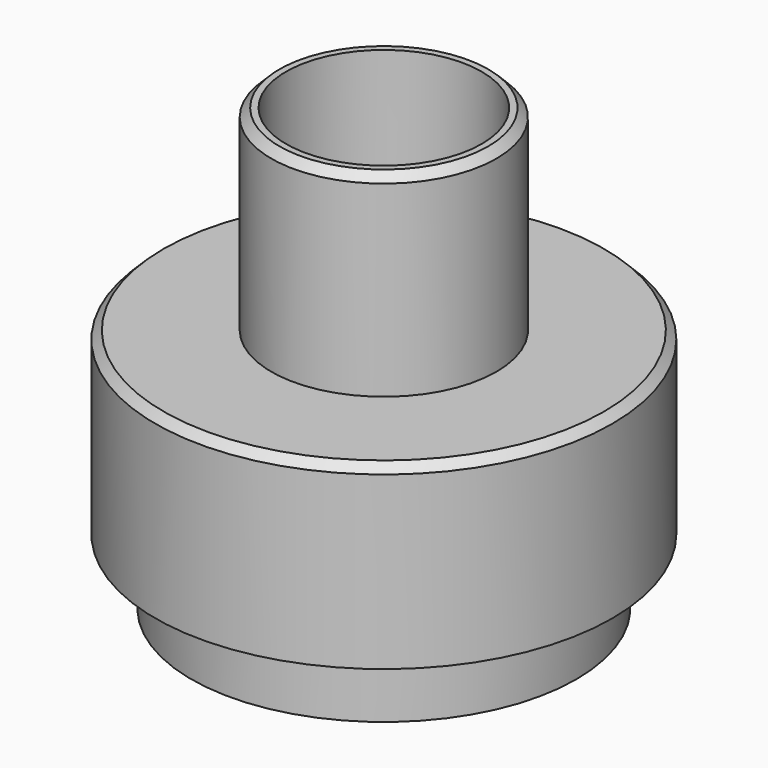
from build123d import *

# Parameters (mm, degrees)
F0_R        = 7
F1_DEPTH    = 5.5
F2_R        = 3.45
F3_DEPTH    = 6
F4_R        = 3
F5_DEPTH    = 25
F6_R        = 6
F6_R_2      = 3
F7_DEPTH    = 2
F8_S5_R     = 6
F8_T6_DEPTH = 11
F9_SIZE     = 0.25
F10_R       = 5.9
F11_DEPTH   = 2
F12_W       = 0.6
F12_H       = 0.6
F13_DEPTH   = 25


# Not quite as in the source:
# - a fillet or chamfer that OpenCascade refuses, or shapes differently, is made with other operations: its cross-section is extruded or revolved along the edge and cut away or added


with BuildPart() as f1:
    # F0 (on Top) → F1 (new body)
    with BuildSketch(Plane.XY):
        Circle(F0_R)
    extrude(amount=F1_DEPTH)

    # F2 (on face) → F3 (join)
    with BuildSketch(Plane.XY.offset(5.5)):
        Circle(F2_R)
    extrude(amount=F3_DEPTH)

    # F4 (on face) → F5 (cut)
    with BuildSketch(Plane.XY.offset(11.5)):
        Circle(F4_R)
    extrude(amount=-F5_DEPTH, mode=Mode.SUBTRACT)

    # F6 (on face) → F7 (cut)
    with BuildSketch(Plane(origin=(0, 0, 0), x_dir=(1, 0, 0), z_dir=(0, 0, -1))):
        Circle(F6_R)
        Circle(F6_R_2, mode=Mode.SUBTRACT)
    extrude(amount=-F7_DEPTH, mode=Mode.SUBTRACT)

    # F8: chamfer of 3.3 on 1 edges, made by hand


with BuildPart() as f8_tool2:
    # F8_s3 → F8_t4 (revolve)
    with BuildSketch(Plane.XZ):
        Polygon((6.3, 2), (3, 5.3), (3, 2), align=None)
    revolve(axis=Axis((0, 0, 2), (0, 0, -1)))

    # F8_s5 → F8_t6 (intersect, symmetric)
    with BuildSketch(Plane.XY.offset(3.6)):
        Circle(F8_S5_R)
    extrude(amount=F8_T6_DEPTH, both=True, mode=Mode.INTERSECT)


with BuildPart() as f1_1:
    add(f1.part)

    # F8_t1: cut F8_tool2
    add(f8_tool2.part, mode=Mode.SUBTRACT)

    # F9
    f9_edges = [f1_1.edges().sort_by_distance(p)[0] for p in [
        (-3.45, 0, 11.5),
        (-7, 0, 5.5),
    ]]
    chamfer(f9_edges, length=F9_SIZE)


with BuildPart() as f11:
    # F10 (on Top) → F11 (new body)
    with BuildSketch(Plane.XY):
        Circle(F10_R)
    extrude(amount=-F11_DEPTH)

    # F12 (on face) → F13 (cut)
    with BuildSketch(Plane(origin=(0, 0, -2), x_dir=(1, 0, 0), z_dir=(0, 0, -1))):
        with Locations((-2.8, 1.4)):
            Rectangle(F12_W, F12_H)
        with Locations((-2.8, 2.8)):
            Rectangle(F12_W, F12_H)
        with Locations((-2.8, 4.2)):
            Rectangle(F12_W, F12_H)
        with Locations((-1.4, 4.2)):
            Rectangle(F12_W, F12_H)
        with Locations((0, 4.2)):
            Rectangle(F12_W, F12_H)
        with Locations((1.4, 4.2)):
            Rectangle(F12_W, F12_H)
        with Locations((-4.2, 2.8)):
            Rectangle(F12_W, F12_H)
        with Locations((-4.2, 1.4)):
            Rectangle(F12_W, F12_H)
        with Locations((-4.2, 0)):
            Rectangle(F12_W, F12_H)
        with Locations((-4.2, -1.4)):
            Rectangle(F12_W, F12_H)
        with Locations((-4.2, -2.8)):
            Rectangle(F12_W, F12_H)
        with Locations((-2.8, -2.8)):
            Rectangle(F12_W, F12_H)
        with Locations((-2.8, -1.4)):
            Rectangle(F12_W, F12_H)
        with Locations((-2.8, 0)):
            Rectangle(F12_W, F12_H)
        with Locations((-1.4, 1.4)):
            Rectangle(F12_W, F12_H)
        with Locations((-1.4, 2.8)):
            Rectangle(F12_W, F12_H)
        with Locations((0, 2.8)):
            Rectangle(F12_W, F12_H)
        with Locations((0, 1.4)):
            Rectangle(F12_W, F12_H)
        Rectangle(F12_W, F12_H)
        with Locations((-1.4, 0)):
            Rectangle(F12_W, F12_H)
        with Locations((-1.4, -1.4)):
            Rectangle(F12_W, F12_H)
        with Locations((-1.4, -2.8)):
            Rectangle(F12_W, F12_H)
        with Locations((-2.8, -4.2)):
            Rectangle(F12_W, F12_H)
        with Locations((-1.4, -4.2)):
            Rectangle(F12_W, F12_H)
        with Locations((0, -4.2)):
            Rectangle(F12_W, F12_H)
        with Locations((1.4, -4.2)):
            Rectangle(F12_W, F12_H)
        with Locations((2.8, -4.2)):
            Rectangle(F12_W, F12_H)
        with Locations((4.2, -2.8)):
            Rectangle(F12_W, F12_H)
        with Locations((2.8, -2.8)):
            Rectangle(F12_W, F12_H)
        with Locations((1.4, -2.8)):
            Rectangle(F12_W, F12_H)
        with Locations((1.4, -1.4)):
            Rectangle(F12_W, F12_H)
        with Locations((1.4, 0)):
            Rectangle(F12_W, F12_H)
        with Locations((1.4, 1.4)):
            Rectangle(F12_W, F12_H)
        with Locations((2.8, 4.2)):
            Rectangle(F12_W, F12_H)
        with Locations((4.2, 2.8)):
            Rectangle(F12_W, F12_H)
        with Locations((4.2, 1.4)):
            Rectangle(F12_W, F12_H)
        with Locations((4.2, 0)):
            Rectangle(F12_W, F12_H)
        with Locations((4.2, -1.4)):
            Rectangle(F12_W, F12_H)
        with Locations((2.8, -1.4)):
            Rectangle(F12_W, F12_H)
        with Locations((2.8, 0)):
            Rectangle(F12_W, F12_H)
        with Locations((2.8, 1.4)):
            Rectangle(F12_W, F12_H)
        with Locations((2.8, 2.8)):
            Rectangle(F12_W, F12_H)
        with Locations((0, -1.4)):
            Rectangle(F12_W, F12_H)
        with Locations((0, -2.8)):
            Rectangle(F12_W, F12_H)
        with Locations((1.4, 2.8)):
            Rectangle(F12_W, F12_H)
    extrude(amount=-F13_DEPTH, mode=Mode.SUBTRACT)


solid = Compound([f1_1.part, f11.part])
